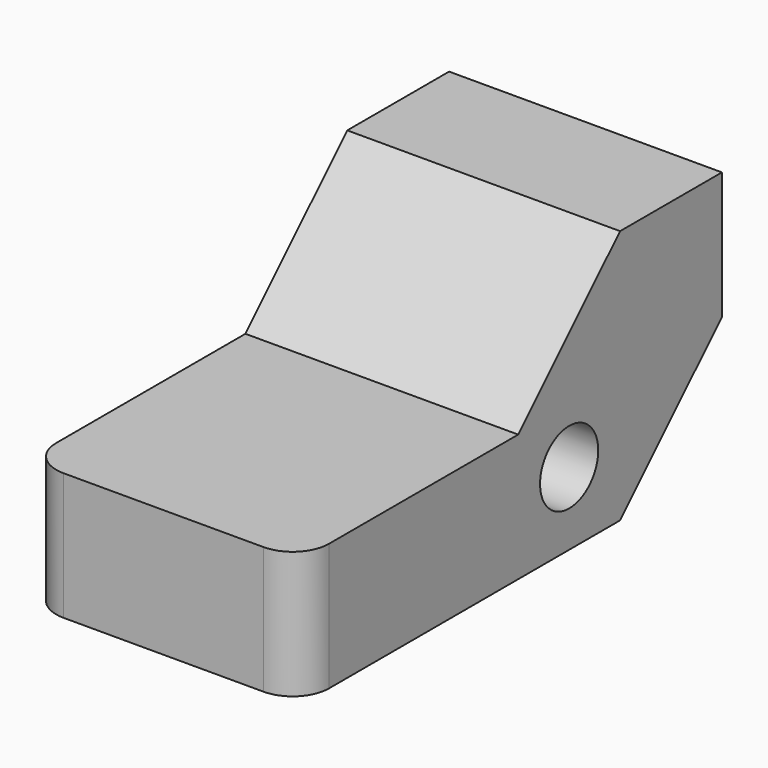
from build123d import *

# Parameters (mm, degrees)
F2_DEPTH = 35.56
F0_R     = 10.16
F3_DEPTH = 76.2


# Not quite as in the source:
# - a feature names something its author has since deleted; it is built from what else it names


with BuildPart() as f2:
    # F1 (on Top) → F2 (new body)
    with BuildSketch(Plane.XY):
        with BuildLine():
            Line((0, 76.2), (-76.2, 76.2))
            Line((-76.2, 76.2), (-76.2, 10.16))
            ThreePointArc((-76.2, 10.16), (-73.2242048969, 2.9757951031), (-66.04, 0))
            Line((-66.04, 0), (-10.16, 0))
            ThreePointArc((-10.16, 0), (-2.9757951031, 2.9757951031), (0, 10.16))
            Line((0, 10.16), (0, 76.2))
        make_face()
    extrude(amount=F2_DEPTH)

    # F0 (on Right) → F3 (join)
    with BuildSketch(Plane.YZ):
        Polygon((76.2, 0), (111.76, 0), (147.32, 35.56), (147.32, 71.12), (111.76, 71.12), (76.2, 35.56), align=None)
        with Locations((93.98, 20.32)):
            Circle(F0_R, mode=Mode.SUBTRACT)
    extrude(amount=-F3_DEPTH)


solid = f2.part
